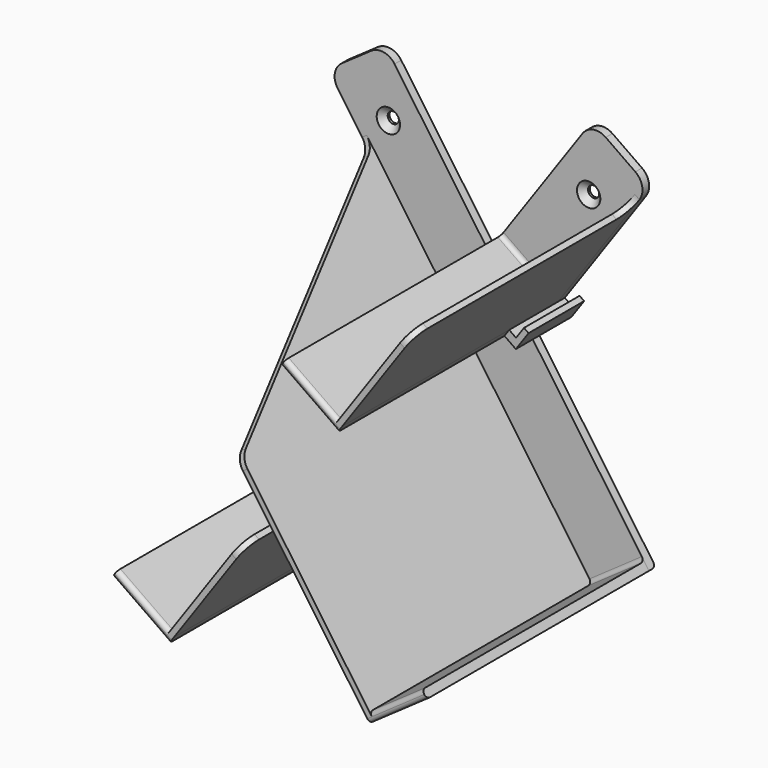
from build123d import *

# Parameters (mm, degrees)
F0_R          = 2
F1_DEPTH      = 3
F4_DEPTH      = 2
F3_W          = 100
F3_H          = 3
F5_DEPTH      = 25
F6_DEPTH      = 25
F7_DEPTH      = 100
F9_W          = 97
F9_H          = 45
F10_DEPTH     = 2
F11_R         = 5.99999
F12_T1_DEPTH  = 23
F12_T3_DEPTH  = 25
F12_T5_DEPTH  = 23
F12_T7_DEPTH  = 25
F12_T9_DEPTH  = 32.5
F12_T11_DEPTH = 26.75
F12_T13_DEPTH = 32.5
F12_T15_DEPTH = 26.75
F12_T17_DEPTH = 37.5
F12_T19_DEPTH = 37.5
F12_T21_DEPTH = 32.5
F13_R         = 0.99999
F14_SIZE      = 2.2


# Not quite as in the source:
# - a fillet or chamfer that OpenCascade refuses, or shapes differently, is made with other operations: its cross-section is extruded or revolved along the edge and cut away or added
# - a fillet or chamfer is up to 0.001 mm smaller than in the source, because OpenCascade refuses the exact size
# - a feature names something its author has since deleted; it is built from what else it names


with BuildPart() as f1:
    # F0 (on Front) → F1 (new body)
    with BuildSketch(Plane.XZ):
        Polygon((-15.2596823595, 0), (0, 21.7930849453), (-37.2558830062, 75), (-57.7346841134, 60.6605890912), align=None)
        with Locations((-36.0237548328, 51.4472536598)):
            Circle(F0_R, mode=Mode.SUBTRACT)
        Polygon((0, -21.7930849453), (15.2596823595, 0), (0, 21.7930849453), (-15.2596823595, 0), align=None)
        Polygon((25.0408272414, 13.9689225668), (57.7346841134, 60.6605890912), (37.2558830062, 75), (4.5620261342, 28.3083334755), align=None)
        with Locations((36.0237548328, 51.4472536598)):
            Circle(F0_R, mode=Mode.SUBTRACT)
        Polygon((15.2596823595, 0), (23.3200979324, 11.5114664339), (2.8412968251, 25.8508773427), (0, 21.7930849453), align=None)
        Polygon((23.3200979324, 11.5114664339), (25.0408272414, 13.9689225668), (4.5620261342, 28.3083334755), (2.8412968251, 25.8508773427), align=None)
        Polygon((-35.5351536972, -72.5425438671), (0, -21.7930849453), (-15.2596823595, 0), (-56.0139548044, -58.2031329584), align=None)
        Polygon((57.7346841134, -60.6605890912), (15.2596823595, 0), (0, -21.7930849453), (35.5351536972, -72.5425438671), (37.2558830062, -75), align=None)
        Polygon((-37.2558830062, -75), (-35.5351536972, -72.5425438671), (-56.0139548044, -58.2031329584), (-57.7346841134, -60.6605890912), align=None)
    extrude(amount=F1_DEPTH)

    # F3 (on offset) → F4 (join)
    with BuildSketch(Plane(origin=(-10.2394005536, 0, -7.1697054544), x_dir=(0, -1, 0), z_dir=(-0.8191520443, 0, -0.5735764364))):
        Polygon((3, -79.8054999295), (103, -79.8054999295), (103, 0.1945000705), (83, 0.1945000705), (90.1471648731, -3.9319174929), (90.1471648731, -52.514305784), (48.0735824366, -76.8054999295), (6, -52.514305784), (6, -3.9319174929), (13.1471648731, 0.1945000705), (3, 0.1945000705), align=None)
        Polygon((83, 0.1945000705), (103, 0.1945000705), (3, 57.9295269895), (3, 0.1945000705), (13.1471648731, 0.1945000705), (48.0735824366, 20.3592766526), align=None)
        Polygon((90.1471648731, -3.9319174929), (83, 0.1945000705), (13.1471648731, 0.1945000705), (6, -3.9319174929), (6, -52.514305784), (48.0735824366, -76.8054999295), (90.1471648731, -52.514305784), align=None)
        Polygon((13.1471648731, 0.1945000705), (83, 0.1945000705), (48.0735824366, 20.3592766526), align=None)
    extrude(amount=-F4_DEPTH)

    # F3 (on offset) → F5 (join)
    with BuildSketch(Plane(origin=(-10.2394005536, 0, -7.1697054544), x_dir=(0, -1, 0), z_dir=(-0.8191520443, 0, -0.5735764364))):
        with Locations((53, -81.3054999295)):
            Rectangle(F3_W, F3_H)
    extrude(amount=-F5_DEPTH)

    # F0 (on Front) → F6 (join)
    with BuildSketch(Plane.XZ):
        Polygon((-33.0776975643, -74.2632731762), (-35.5351536972, -72.5425438671), (-37.2558830062, -75), (-33.1601227848, -77.8678821818), (-28.571511294, -71.3146658274), (-30.2098153825, -70.1675129547), align=None)
        Polygon((37.2558830062, -75), (35.5351536972, -72.5425438671), (33.0776975643, -74.2632731762), (30.2098153825, -70.1675129547), (28.571511294, -71.3146658274), (33.1601227848, -77.8678821818), align=None)
        Polygon((27.4982833743, 12.2481932577), (25.0408272414, 13.9689225668), (23.3200979324, 11.5114664339), (27.4158581538, 8.6435842521), (32.0044696446, 15.1968006064), (30.366165556, 16.3439534791), align=None)
    extrude(amount=F6_DEPTH)

    # F0 (on Front) → F7 (join)
    with BuildSketch(Plane.XZ):
        Polygon((-37.2558830062, -75), (-35.5351536972, -72.5425438671), (-56.0139548044, -58.2031329584), (-57.7346841134, -60.6605890912), align=None)
        Polygon((23.3200979324, 11.5114664339), (25.0408272414, 13.9689225668), (4.5620261342, 28.3083334755), (2.8412968251, 25.8508773427), align=None)
    extrude(amount=F7_DEPTH)

    # F9 (on offset) → F10 (join)
    with BuildSketch(Plane(origin=(10.2394005536, 0, -7.1697054544), x_dir=(0, 1, 0), z_dir=(0.8191520443, 0, -0.5735764364))):
        with Locations((-51.5, -57.3054999295)):
            Rectangle(F9_W, F9_H)
        Polygon((-94, -57.3054999295), (-84.4737205584, -40.8054999295), (-65.4211616751, -40.8054999295), (-55.8948822335, -57.3054999295), (-65.4211616751, -73.8054999295), (-84.4737205584, -73.8054999295), align=None, mode=Mode.SUBTRACT)
        Polygon((-9, -57.3054999295), (-18.5262794416, -73.8054999295), (-37.5788383249, -73.8054999295), (-47.1051177665, -57.3054999295), (-37.5788383249, -40.8054999295), (-18.5262794416, -40.8054999295), align=None, mode=Mode.SUBTRACT)
        with Locations((-51.5, 48.3054999295)):
            Rectangle(F9_W, F9_H)
        Polygon((-55.8948822335, 48.3054999295), (-65.4211616751, 31.8054999295), (-84.4737205584, 31.8054999295), (-94, 48.3054999295), (-84.4737205584, 64.8054999295), (-65.4211616751, 64.8054999295), align=None, mode=Mode.SUBTRACT)
        Polygon((-9, 48.3054999295), (-18.5262794416, 31.8054999295), (-37.5788383249, 31.8054999295), (-47.1051177665, 48.3054999295), (-37.5788383249, 64.8054999295), (-18.5262794416, 64.8054999295), align=None, mode=Mode.SUBTRACT)
        Polygon((-84.4737205584, 31.8054999295), (-65.4211616751, 31.8054999295), (-55.8948822335, 48.3054999295), (-65.4211616751, 64.8054999295), (-84.4737205584, 64.8054999295), (-94, 48.3054999295), align=None)
        Polygon((-37.5788383249, 31.8054999295), (-18.5262794416, 31.8054999295), (-9, 48.3054999295), (-18.5262794416, 64.8054999295), (-37.5788383249, 64.8054999295), (-47.1051177665, 48.3054999295), align=None)
        Polygon((-65.4211616751, -40.8054999295), (-84.4737205584, -40.8054999295), (-94, -57.3054999295), (-84.4737205584, -73.8054999295), (-65.4211616751, -73.8054999295), (-55.8948822335, -57.3054999295), align=None)
        Polygon((-37.5788383249, -73.8054999295), (-18.5262794416, -73.8054999295), (-9, -57.3054999295), (-18.5262794416, -40.8054999295), (-37.5788383249, -40.8054999295), (-47.1051177665, -57.3054999295), align=None)
    extrude(amount=-F10_DEPTH)

    # F11 (radius 6 in the source; OpenCascade refuses exactly that, so slightly less here)
    f11_edges = [f1.edges().sort_by_distance(p)[0] for p in [
        (-10.543366, -3, -35.107125),
        (-10.543366, -100, -35.107125),
        (50.032615, -100, 51.404341),
        (50.032615, -3, 51.404341),
        (-42.64726, -3, 40.856961),
        (-9.531809, -103, -6.436804),
        (-57.734684, -1.5, 60.660589),
        (-37.255883, -1.5, 75),
        (37.255883, -1.5, 75),
        (57.734684, -1.5, 60.660589),
    ]]
    fillet(f11_edges, radius=F11_R)

    # F12: fillet of radius 1.5 on 18 edges, made by hand

    # F12_s2 → F12_t1 (join)
    with BuildSketch(Plane(origin=(-10.2394005536, 0, 7.1697054544), x_dir=(0, 1, 0), z_dir=(0.8191520443, 0, -0.5735764364))):
        with BuildLine():
            ThreePointArc((-3, 27.3054999295), (-3.4393398282, 26.2448397577), (-4.5, 25.8054999295))
            Line((-4.5, 25.8054999295), (-3, 25.8054999295))
            Line((-3, 25.8054999295), (-3, 27.3054999295))
        make_face()
        with BuildLine():
            ThreePointArc((-3, -78.3054999295), (-3.4393398282, -79.3661601013), (-4.5, -79.8054999295))
            Line((-4.5, -79.8054999295), (-3, -79.8054999295))
            Line((-3, -79.8054999295), (-3, -78.3054999295))
        make_face()
    extrude(amount=F12_T1_DEPTH)

    # F12_s4 → F12_t3 (join)
    with BuildSketch(Plane(origin=(10.2394005536, 0, -7.1697054544), x_dir=(0, 1, 0), z_dir=(-0.8191520443, 0, 0.5735764364))):
        with BuildLine():
            ThreePointArc((-3, -21.3054999295), (-3.4393398282, -22.3661601013), (-4.5, -22.8054999295))
            Line((-4.5, -22.8054999295), (-3, -22.8054999295))
            Line((-3, -22.8054999295), (-3, -21.3054999295))
        make_face()
    extrude(amount=F12_T3_DEPTH)

    # F12_s6 → F12_t5 (join)
    with BuildSketch(Plane(origin=(-8.601096465, 0, -6.0225525817), x_dir=(0, 1, 0), z_dir=(0.8191520443, 0, 0.5735764364))):
        with BuildLine():
            ThreePointArc((-3, -78.3054999295), (-3.4393398282, -79.3661601013), (-4.5, -79.8054999295))
            Line((-4.5, -79.8054999295), (-3, -79.8054999295))
            Line((-3, -79.8054999295), (-3, -78.3054999295))
        make_face()
    extrude(amount=F12_T5_DEPTH)

    # F12_s8 → F12_t7 (join)
    with BuildSketch(Plane.XZ):
        with BuildLine():
            ThreePointArc((34.6747890426, -71.3138158007), (34.9232726057, -72.4346527217), (34.3064256307, -73.4029085217))
            Line((34.3064256307, -73.4029085217), (35.5351536972, -72.5425438671))
            Line((35.5351536972, -72.5425438671), (34.6747890426, -71.3138158007))
        make_face()
        with BuildLine():
            ThreePointArc((-32.2173329098, -73.0345451098), (-33.1855887097, -73.6513920847), (-34.3064256307, -73.4029085217))
            Line((-34.3064256307, -73.4029085217), (-33.0776975643, -74.2632731762))
            Line((-33.0776975643, -74.2632731762), (-32.2173329098, -73.0345451098))
        make_face()
        with BuildLine():
            ThreePointArc((-34.3064256307, -73.4029085217), (-34.9232726057, -72.4346527217), (-34.6747890426, -71.3138158007))
            Line((-34.6747890426, -71.3138158007), (-35.5351536972, -72.5425438671))
            Line((-35.5351536972, -72.5425438671), (-34.3064256307, -73.4029085217))
        make_face()
        with BuildLine():
            ThreePointArc((34.3064256307, -73.4029085217), (33.1855887097, -73.6513920847), (32.2173329098, -73.0345451098))
            Line((32.2173329098, -73.0345451098), (33.0776975643, -74.2632731762))
            Line((33.0776975643, -74.2632731762), (34.3064256307, -73.4029085217))
        make_face()
    extrude(amount=F12_T7_DEPTH)

    # F12_s10 → F12_t9 (cut)
    with BuildSketch(Plane(origin=(-13.3112207197, 0, 9.3206170907), x_dir=(0, 1, 0), z_dir=(0.8191520443, 0, -0.5735764364))):
        with BuildLine():
            ThreePointArc((-98.5, -82.8054999295), (-99.5606601718, -82.3661601013), (-100, -81.3054999295))
            Line((-100, -81.3054999295), (-100, -82.8054999295))
            Line((-100, -82.8054999295), (-98.5, -82.8054999295))
        make_face()
        with BuildLine():
            ThreePointArc((-98.5, 22.8054999295), (-99.5606601718, 23.2448397577), (-100, 24.3054999295))
            Line((-100, 24.3054999295), (-100, 22.8054999295))
            Line((-100, 22.8054999295), (-98.5, 22.8054999295))
        make_face()
    extrude(amount=F12_T9_DEPTH, mode=Mode.SUBTRACT)

    # F12_s12 → F12_t11 (cut)
    with BuildSketch(Plane(origin=(8.601096465, 0, -6.0225525817), x_dir=(0, 1, 0), z_dir=(-0.8191520443, 0, 0.5735764364))):
        with BuildLine():
            ThreePointArc((-100, -24.3054999295), (-99.5606601718, -25.3661601013), (-98.5, -25.8054999295))
            Line((-98.5, -25.8054999295), (-100, -25.8054999295))
            Line((-100, -25.8054999295), (-100, -24.3054999295))
        make_face()
        with BuildLine():
            ThreePointArc((-100, 81.3054999295), (-99.5606601718, 80.2448397577), (-98.5, 79.8054999295))
            Line((-98.5, 79.8054999295), (-100, 79.8054999295))
            Line((-100, 79.8054999295), (-100, 81.3054999295))
        make_face()
    extrude(amount=F12_T11_DEPTH, mode=Mode.SUBTRACT)

    # F12_s14 → F12_t13 (cut)
    with BuildSketch(Plane(origin=(-13.3112207197, 0, -9.3206170907), x_dir=(0, 1, 0), z_dir=(0.8191520443, 0, 0.5735764364))):
        with BuildLine():
            ThreePointArc((-103, -81.3054999295), (-102.5606601718, -82.3661601013), (-101.5, -82.8054999295))
            Line((-101.5, -82.8054999295), (-103, -82.8054999295))
            Line((-103, -82.8054999295), (-103, -81.3054999295))
        make_face()
    extrude(amount=F12_T13_DEPTH, mode=Mode.SUBTRACT)

    # F12_s16 → F12_t15 (cut)
    with BuildSketch(Plane(origin=(-8.601096465, 0, -6.0225525817), x_dir=(0, 1, 0), z_dir=(0.8191520443, 0, 0.5735764364))):
        with BuildLine():
            ThreePointArc((-101.5, -79.8054999295), (-102.5606601718, -80.2448397577), (-103, -81.3054999295))
            Line((-103, -81.3054999295), (-103, -79.8054999295))
            Line((-103, -79.8054999295), (-101.5, -79.8054999295))
        make_face()
    extrude(amount=F12_T15_DEPTH, mode=Mode.SUBTRACT)

    # F12_s18 → F12_t17 (cut)
    with BuildSketch(Plane(origin=(17.4069809411, 0, -12.1884992725), x_dir=(0, 1, 0), z_dir=(-0.8191520443, 0, 0.5735764364))):
        with BuildLine():
            ThreePointArc((-1.5, 82.8054999295), (-0.4393398282, 82.3661601013), (0, 81.3054999295))
            Line((0, 81.3054999295), (0, 82.8054999295))
            Line((0, 82.8054999295), (-1.5, 82.8054999295))
        make_face()
    extrude(amount=F12_T17_DEPTH, mode=Mode.SUBTRACT)

    # F12_s20 → F12_t19 (cut)
    with BuildSketch(Plane(origin=(13.3112207197, 0, 9.3206170907), x_dir=(0, 1, 0), z_dir=(-0.8191520443, 0, -0.5735764364))):
        with BuildLine():
            ThreePointArc((-1.5, 82.8054999295), (-0.4393398282, 82.3661601013), (0, 81.3054999295))
            Line((0, 81.3054999295), (0, 82.8054999295))
            Line((0, 82.8054999295), (-1.5, 82.8054999295))
        make_face()
    extrude(amount=F12_T19_DEPTH, mode=Mode.SUBTRACT)

    # F12_s22 → F12_t21 (cut)
    with BuildSketch(Plane.XZ.offset(-3.75)):
        with BuildLine():
            ThreePointArc((34.3888508512, -77.0075175272), (33.2680139302, -77.2560010903), (32.2997581302, -76.6391541153))
            Line((32.2997581302, -76.6391541153), (33.1601227848, -77.8678821818))
            Line((33.1601227848, -77.8678821818), (34.3888508512, -77.0075175272))
        make_face()
        with BuildLine():
            ThreePointArc((-34.3888508512, -77.0075175272), (-33.2680139302, -77.2560010903), (-32.2997581302, -76.6391541153))
            Line((-32.2997581302, -76.6391541153), (-33.1601227848, -77.8678821818))
            Line((-33.1601227848, -77.8678821818), (-34.3888508512, -77.0075175272))
        make_face()
    extrude(amount=F12_T21_DEPTH, mode=Mode.SUBTRACT)

    # F13 (radius 1 in the source; OpenCascade refuses exactly that, so slightly less here)
    f13_edges = [f1.edges().sort_by_distance(p)[0] for p in [
        (-28.571511, -12.5, -71.314666),
        (28.571511, -12.5, -71.314666),
        (-30.209815, -12.5, -70.167513),
        (30.209815, -12.5, -70.167513),
    ]]
    fillet(f13_edges, radius=F13_R)

    # F14
    f14_edges = [f1.edges().sort_by_distance(p)[0] for p in [
        (-38.023755, -3, 51.447254),
        (34.023755, -3, 51.447254),
    ]]
    chamfer(f14_edges, length=F14_SIZE)


solid = f1.part
